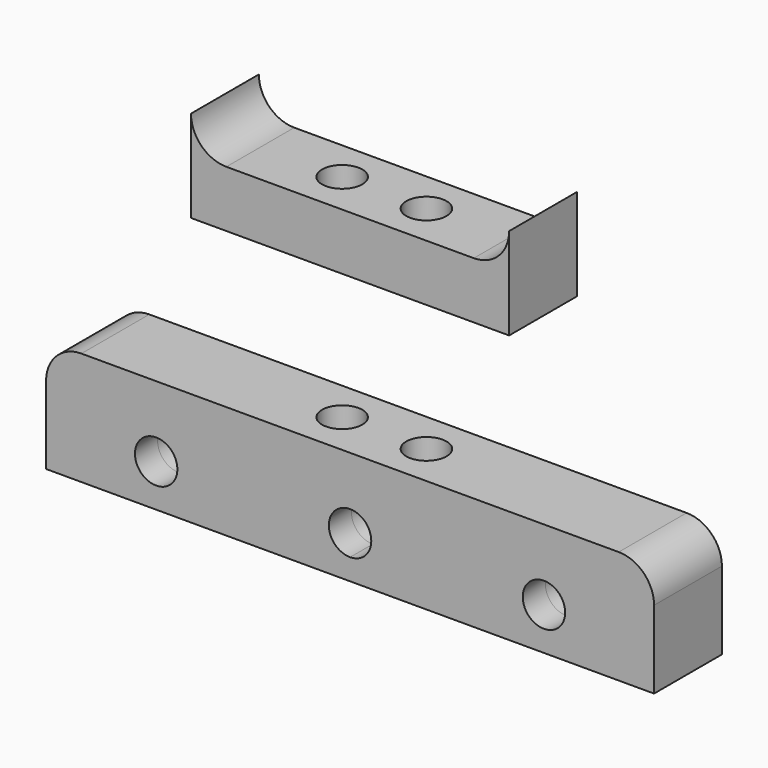
from build123d import *

# Parameters (mm, degrees)
F0_R          = 2.85
F1_DEPTH      = 16
F2_R          = 3
F3_DEPTH      = 12.5
F5_DEPTH      = 40
F7_DEPTH      = 8
F7_DEPTH_BACK = 4
F8_DEPTH      = 50.929265815
F9_R          = 5


# Not quite as in the source:
# - a feature names something its author has since deleted; it is built from what else it names


with BuildPart() as f1:
    # F0 (on Top) → F1 (new body)
    with BuildSketch(Plane.XY):
        Polygon((20.2244706452, -4), (35, -4), (43, -4), (43, 8), (35, 8), (20.2244706452, 8), (19.8490470648, 8), (-35, 8), (-43, 8), (-43, -4), (-35, -4), (-20.2244706452, -4), (-19.8490470648, -4), (19.8490470648, -4), align=None)
        with Locations((-6.0009112008, 2.1045637578)):
            Circle(F0_R, mode=Mode.SUBTRACT)
        with Locations((6, 2)):
            Circle(F0_R, mode=Mode.SUBTRACT)
    extrude(amount=F1_DEPTH)

    # F2 (on Front) → F3 (cut, symmetric)
    with BuildSketch(Plane.XZ):
        with Locations((-27.4271778762, 6)):
            Circle(F2_R)
        with Locations((27.4271778762, 6)):
            Circle(F2_R)
        with BuildLine():
            ThreePointArc((0, 9), (-3, 6), (0, 3))
            Line((0, 3), (0, 9))
        make_face()
        with BuildLine():
            Line((0, 9), (0, 3))
            ThreePointArc((0, 3), (2.1213203436, 3.8786796564), (3, 6))
            ThreePointArc((3, 6), (2.1213203436, 8.1213203436), (0, 9))
        make_face()
    extrude(amount=F3_DEPTH, both=True, mode=Mode.SUBTRACT)

    # F4 (on Right) → F5 (cut, symmetric)
    with BuildSketch(Plane.YZ):
        with BuildLine():
            ThreePointArc((0, 10.5), (1.0606601718, 10.9393398282), (1.5, 12))
            ThreePointArc((1.5, 12), (-1.0606601718, 13.0606601718), (0, 10.5))
        make_face()
    extrude(amount=F5_DEPTH, both=True, mode=Mode.SUBTRACT)

    # F9
    f9_edges = [f1.edges().sort_by_distance(p)[0] for p in [
        (-43, 2, 16),
        (43, 2, 16),
    ]]
    fillet(f9_edges, radius=F9_R)


with BuildPart() as f7:
    # F6 (on Front) → F7 (new body, two sides)
    with BuildSketch(Plane.XZ) as f7_sk:
        with BuildLine():
            Line((-22.5, 50.928265815), (-22.5, 37.928265815))
            Line((-22.5, 37.928265815), (22.5, 37.928265815))
            Line((22.5, 37.928265815), (22.5, 45.928265815))
            Line((22.5, 45.928265815), (22.5, 50.928265815))
            ThreePointArc((22.5, 50.928265815), (21.0355339059, 47.3927319091), (17.5, 45.928265815))
            Line((17.5, 45.928265815), (-17.5, 45.928265815))
            ThreePointArc((-17.5, 45.928265815), (-21.0355339059, 47.3927319091), (-22.5, 50.928265815))
        make_face()
    extrude(amount=-F7_DEPTH)
    extrude(f7_sk.sketch, amount=F7_DEPTH_BACK)

    # F0 (on Top) → F8 (cut, through all)
    with BuildSketch(Plane.XY):
        with Locations((-6.0009112008, 2.1045637578)):
            Circle(F0_R)
        with Locations((6, 2)):
            Circle(F0_R)
    extrude(amount=F8_DEPTH, mode=Mode.SUBTRACT)


solid = Compound([f1.part, f7.part])
